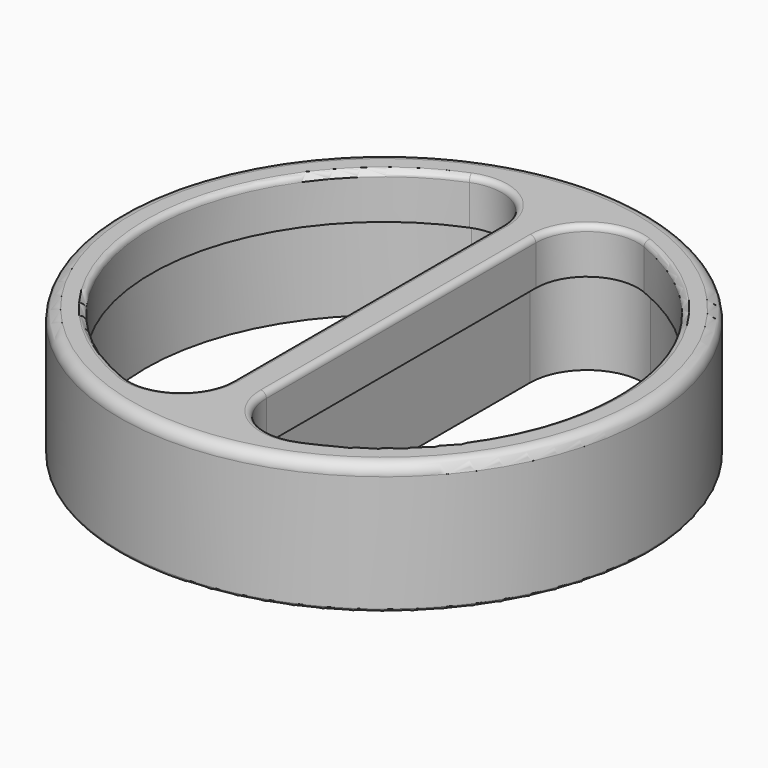
from build123d import *

# Parameters (mm, degrees)
F0_R     = 46.5
F1_DEPTH = 23
F3_DEPTH = 15
F4_R     = 1
F5_R     = 45
F5_R_2   = 44
F6_DEPTH = 20
F7_R     = 0.5
F8_R     = 2


# Not quite as in the source:
# - a feature names something its author has since deleted; it is built from what else it names


with BuildPart() as f1:
    # F0 (on Top) → F1 (new body)
    with BuildSketch(Plane.XY):
        Circle(F0_R)
        with BuildLine():
            ThreePointArc((-15.375, -38.0080172464), (-41, 0), (-15.375, 38.0080172464))
            ThreePointArc((-15.375, 38.0080172464), (-6.9688470506, 37.1271997267), (-3, 29.6647939484))
            Line((-3, 29.6647939484), (-3, -29.6647939484))
            ThreePointArc((-3, -29.6647939484), (-6.9688470506, -37.1271997267), (-15.375, -38.0080172464))
        make_face(mode=Mode.SUBTRACT)
        with BuildLine():
            Line((3, -29.6647939484), (3, 29.6647939484))
            ThreePointArc((3, 29.6647939484), (6.9688470506, 37.1271997267), (15.375, 38.0080172464))
            ThreePointArc((15.375, 38.0080172464), (41, 0), (15.375, -38.0080172464))
            ThreePointArc((15.375, -38.0080172464), (6.9688470506, -37.1271997267), (3, -29.6647939484))
        make_face(mode=Mode.SUBTRACT)
    extrude(amount=-F1_DEPTH)

    # F2 (on face) → F3 (cut)
    with BuildSketch(Plane(origin=(0, 0, -23), x_dir=(1, 0, 0), z_dir=(0, 0, -1))):
        with BuildLine():
            ThreePointArc((-15.75, -38.9350420573), (-6.4098300563, -37.9563559243), (-2, -29.6647939484))
            Line((-2, -29.6647939484), (-2, 29.6647939484))
            ThreePointArc((-2, 29.6647939484), (-6.4098300563, 37.9563559243), (-15.75, 38.9350420573))
            ThreePointArc((-15.75, 38.9350420573), (-42, 0), (-15.75, -38.9350420573))
        make_face()
        with BuildLine():
            Line((-3, 29.6647939484), (-3, -29.6647939484))
            ThreePointArc((-3, -29.6647939484), (-6.9688470506, -37.1271997267), (-15.375, -38.0080172464))
            ThreePointArc((-15.375, -38.0080172464), (-41, 0), (-15.375, 38.0080172464))
            ThreePointArc((-15.375, 38.0080172464), (-6.9688470506, 37.1271997267), (-3, 29.6647939484))
        make_face(mode=Mode.SUBTRACT)
        with BuildLine():
            ThreePointArc((2, -29.6647939484), (6.4098300563, -37.9563559243), (15.75, -38.9350420573))
            ThreePointArc((15.75, -38.9350420573), (42, 0), (15.75, 38.9350420573))
            ThreePointArc((15.75, 38.9350420573), (6.4098300563, 37.9563559243), (2, 29.6647939484))
            Line((2, 29.6647939484), (2, -29.6647939484))
        make_face()
        with BuildLine():
            ThreePointArc((3, 29.6647939484), (6.9688470506, 37.1271997267), (15.375, 38.0080172464))
            ThreePointArc((15.375, 38.0080172464), (41, 0), (15.375, -38.0080172464))
            ThreePointArc((15.375, -38.0080172464), (6.9688470506, -37.1271997267), (3, -29.6647939484))
            Line((3, -29.6647939484), (3, 29.6647939484))
        make_face(mode=Mode.SUBTRACT)
    extrude(amount=-F3_DEPTH, mode=Mode.SUBTRACT)

    # F4
    f4_edges = [f1.edges().sort_by_distance(p)[0] for p in [
        (-41, 0, 0),
        (3, 0, 0),
    ]]
    fillet(f4_edges, radius=F4_R)

    # F5 (on face) → F6 (cut)
    with BuildSketch(Plane(origin=(0, 0, -23), x_dir=(1, 0, 0), z_dir=(0, 0, -1))):
        Circle(F5_R)
        Circle(F5_R_2, mode=Mode.SUBTRACT)
    extrude(amount=-F6_DEPTH, mode=Mode.SUBTRACT)

    # F7
    f7_edges = [f1.edges().sort_by_distance(p)[0] for p in [
        (-44, 0, -23),
        (-46.5, 0, -23),
    ]]
    fillet(f7_edges, radius=F7_R)

    # F8
    f8_edges = [f1.edges().sort_by_distance(p)[0] for p in [
        (-46.5, 0, 0),
    ]]
    fillet(f8_edges, radius=F8_R)


solid = f1.part
